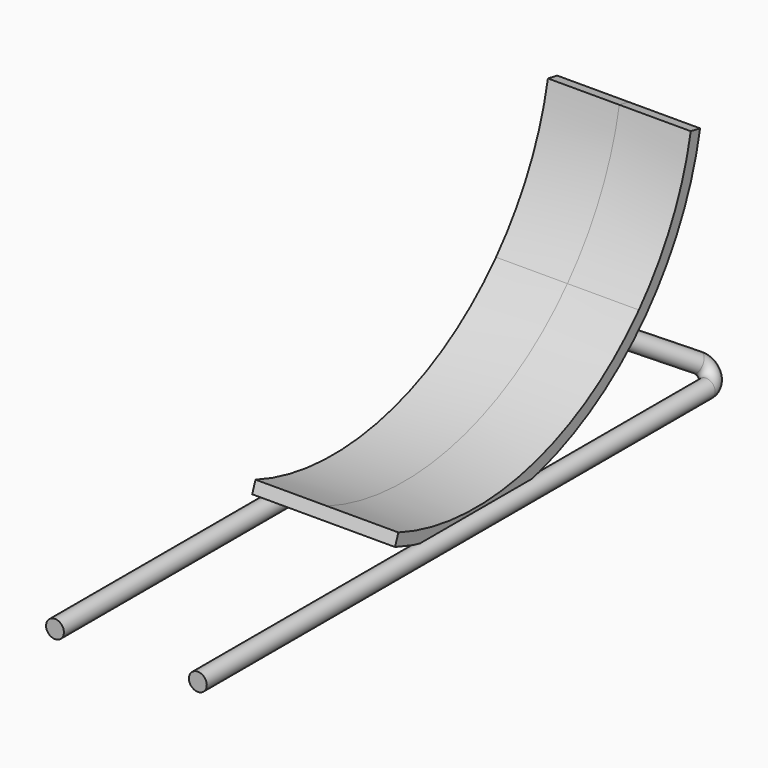
from build123d import *

# Parameters (mm, degrees)
F1_R     = 4.7625
F4_ANGLE = -45
F5_DEPTH = 38.1


with BuildPart() as f2:
    # F2: sweep along a path in F0
    with BuildLine(Plane.YZ) as f2_path:
        Line((-236.3969534289, 0), (102.5836155175, 0))
        ThreePointArc((102.5836155175, 0), (108.5153788964, 4.0835747936), (106.8179141129, 11.0821470185))
        Line((106.8179141129, 11.0821470185), (62.4172823492, 50.8115831453))
    # F1 (on Front) → F2 (sweep)
    with BuildSketch(Plane.XZ):
        Circle(F1_R)
    sweep(path=f2_path.line)


with BuildPart() as f2_1:
    # F4: moved
    add(f2.part.rotate(Axis((0, -66.9066689557, 0), (0, 1, 0)), F4_ANGLE))


with BuildPart() as f5:
    # F3 (on Right) → F5 (new body)
    with BuildSketch(Plane.YZ):
        with BuildLine():
            ThreePointArc((-104.9160923985, 9.8324216778), (-14.9034193722, 4.4089491106), (62.4172823492, 50.8115831453))
            ThreePointArc((62.4172823492, 50.8115831453), (85.4287752957, 84.8267745523), (98.5221539972, 123.7513874376))
            Line((98.5221539972, 123.7513874376), (92.2856373267, 124.9465275208))
            ThreePointArc((92.2856373267, 124.9465275208), (79.7378160711, 87.6437735058), (57.6851353307, 55.0458817407))
            ThreePointArc((57.6851353307, 55.0458817407), (-16.4138704856, 10.5766907908), (-102.6760154692, 15.7741853344))
            Line((-102.6760154692, 15.7741853344), (-104.9160923985, 9.8324216778))
        make_face()
    extrude(amount=-F5_DEPTH)

    # F7: F5 across face


with BuildPart() as f6_1:
    # F6: instance of F2
    add(f2_1.part.mirror(Plane(origin=(-38.1, 12.8891129088, 38.0651309788), x_dir=(0, 1, 0), z_dir=(-1, 0, 0))))


with BuildPart() as f5_1:
    add(f5.part)
    add(f5.part.mirror(Plane(origin=(-38.1, 12.8891129088, 38.0651309788), x_dir=(0, 1, 0), z_dir=(-1, 0, 0))))


solid = Compound([f2_1.part, f6_1.part, f5_1.part])
